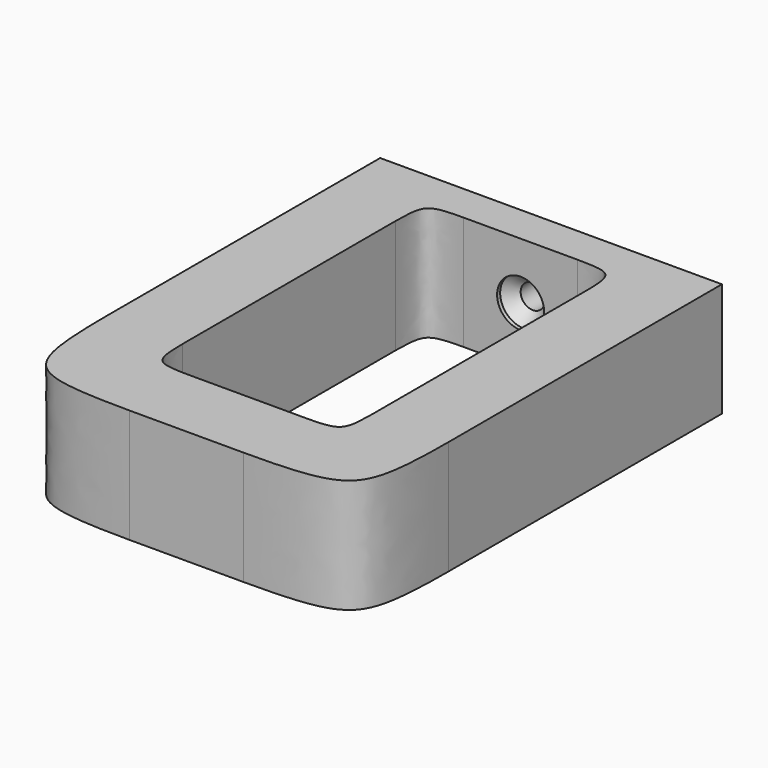
from build123d import *

# Parameters (mm, degrees)
F0_W        = 45
F0_H        = 60
F0_W_2      = 25
F0_H_2      = 45
F1_DEPTH    = 7.5
F4_T1_DEPTH = 15
F5_T1_DEPTH = 90


# Not quite as in the source:
# - a fillet or chamfer that OpenCascade refuses, or shapes differently, is made with other operations: its cross-section is extruded or revolved along the edge and cut away or added


with BuildPart() as f1:
    # F0 (on Top) → F1 (new body, symmetric)
    with BuildSketch(Plane.XY):
        with Locations((0, -30)):
            Rectangle(F0_W, F0_H)
        with Locations((0, -27.5)):
            Rectangle(F0_W_2, F0_H_2, mode=Mode.SUBTRACT)
    extrude(amount=F1_DEPTH, both=True)

    # F2 (on Top) → F3 (revolve, cut)
    with BuildSketch(Plane.XY):
        Polygon((1.6, 0), (0, 0), (0, -5), (3.1, -5), (3.1, -4.5), (1.6, -3), align=None)
    revolve(axis=Axis((0, -2.5, 0), (0, -1, 0)), mode=Mode.SUBTRACT)

    # F4: fillet of radius 5 on 4 edges, made by hand

    # F4_s2 → F4_t1 (join)
    with BuildSketch(Plane.XY.offset(-7.5)):
        with BuildLine():
            add(Edge.make_bspline(
                [(-12.5, -10), (-12.5, -5), (-7.5, -5)],
                knots=[0, 0, 0, 1, 1, 1], degree=2, weights=[1, 2.3333333333, 1]))
            Line((-7.5, -5), (-12.5, -5))
            Line((-12.5, -5), (-12.5, -10))
        make_face()
        with BuildLine():
            add(Edge.make_bspline(
                [(7.5, -5), (12.5, -5), (12.5, -10)],
                knots=[0, 0, 0, 1, 1, 1], degree=2, weights=[1, 2.3333333333, 1]))
            Line((12.5, -10), (12.5, -5))
            Line((12.5, -5), (7.5, -5))
        make_face()
        with BuildLine():
            add(Edge.make_bspline(
                [(-12.5, -45), (-12.5, -50), (-7.5, -50)],
                knots=[0, 0, 0, 1, 1, 1], degree=2, weights=[1, 2.3333333333, 1]))
            Line((-7.5, -50), (-12.5, -50))
            Line((-12.5, -50), (-12.5, -45))
        make_face()
        with BuildLine():
            add(Edge.make_bspline(
                [(12.5, -45), (12.5, -50), (7.5, -50)],
                knots=[0, 0, 0, 1, 1, 1], degree=2, weights=[1, 2.3333333333, 1]))
            Line((7.5, -50), (12.5, -50))
            Line((12.5, -50), (12.5, -45))
        make_face()
    extrude(amount=F4_T1_DEPTH)

    # F5: fillet of radius 15 on 2 edges, made by hand

    # F5_s2 → F5_t1 (cut)
    with BuildSketch(Plane.XY.offset(-45)):
        with BuildLine():
            add(Edge.make_bspline(
                [(-22.5, -45), (-22.5, -60), (-7.5, -60)],
                knots=[0, 0, 0, 1, 1, 1], degree=2, weights=[1, 2.3333333333, 1]))
            Line((-7.5, -60), (-22.5, -60))
            Line((-22.5, -60), (-22.5, -45))
        make_face()
        with BuildLine():
            add(Edge.make_bspline(
                [(22.5, -45), (22.5, -60), (7.5, -60)],
                knots=[0, 0, 0, 1, 1, 1], degree=2, weights=[1, 2.3333333333, 1]))
            Line((7.5, -60), (22.5, -60))
            Line((22.5, -60), (22.5, -45))
        make_face()
    extrude(amount=F5_T1_DEPTH, mode=Mode.SUBTRACT)


solid = f1.part
